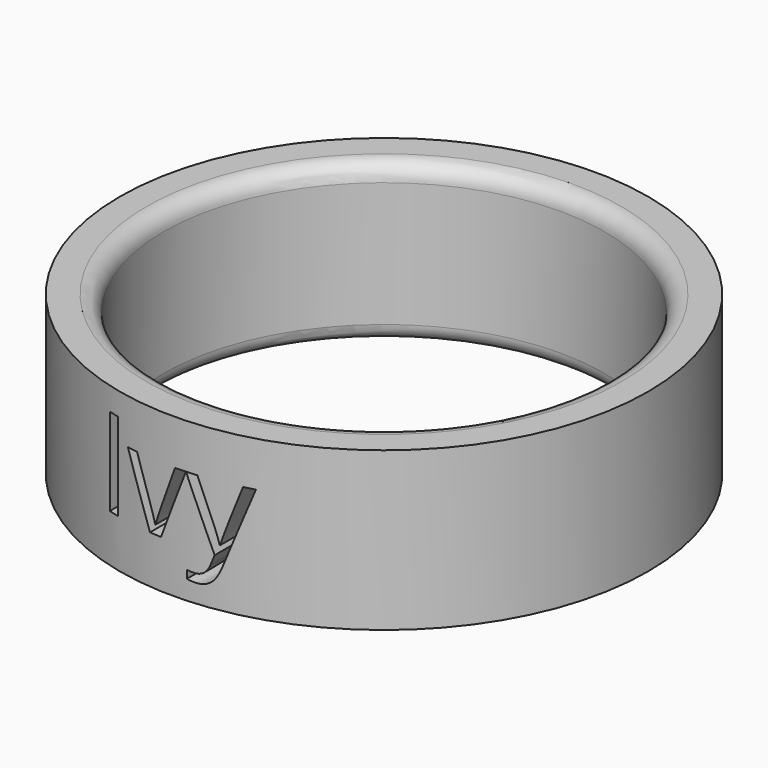
from build123d import *

# Parameters (mm, degrees)
F0_R         = 11.85
F0_R_2       = 9.9
F1_DEPTH     = 7.1
F3_TEXT_SIZE = 5.5006205624
F4_DEPTH     = 10
F5_R         = 0.75


# Not quite as in the source:
# - Text() gives the source's letters only with a copy of the font that has no kerning and outlines rounded to 1/6400 em; it was checked with that copy


with BuildPart() as f1:
    # F0 (on Top) → F1 (new body)
    with BuildSketch(Plane.XY):
        Circle(F0_R)
        Circle(F0_R_2, mode=Mode.SUBTRACT)
    extrude(amount=F1_DEPTH)

    # F3 (on offset) → F4 (cut)
    with BuildSketch(Plane.XZ.offset(11.85)):
        with Locations((-3.7060431039, 2.145928446)):
            Text('Ivy', F3_TEXT_SIZE, font='Open Sans', text_align=(TextAlign.LEFT, TextAlign.BOTTOM))
    extrude(amount=-F4_DEPTH, mode=Mode.SUBTRACT)

    # F5
    f5_edges = [f1.edges().sort_by_distance(p)[0] for p in [
        (-9.9, 0, 7.1),
        (-9.9, 0, 0),
    ]]
    fillet(f5_edges, radius=F5_R)


solid = f1.part
